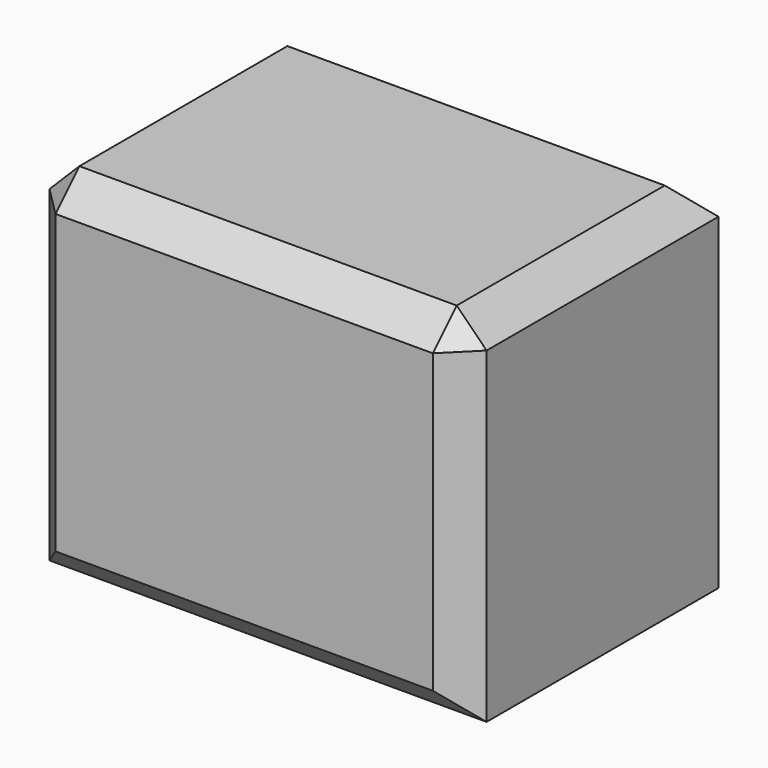
from build123d import *

# Parameters (mm, degrees)
F0_W     = 74.2949992418
F0_H     = 60.6527402997
F1_DEPTH = 54.356
F2_SIZE2 = 5.08
F2_SIZE  = 5.08


# Not quite as in the source:
# - the program builds the solid bodies; features that only make, move or delete a surface that nothing else refers to are left out


with BuildPart() as f1:
    # F0 (on Front) → F1 (new body)
    with BuildSketch(Plane.XZ):
        Rectangle(F0_W, F0_H)
    extrude(amount=F1_DEPTH)

    # F2
    f2_edges = [f1.edges().sort_by_distance(p)[0] for p in [
        (37.1475, -54.356, 0),
        (0, -54.356, 30.32637),
        (-37.1475, -54.356, 0),
        (0, -54.356, -30.32637),
        (37.1475, -27.178, 30.32637),
        (-37.1475, -27.178, 30.32637),
        (0, 0, 30.32637),
    ]]
    chamfer(f2_edges, length=F2_SIZE, length2=F2_SIZE2)


solid = f1.part
